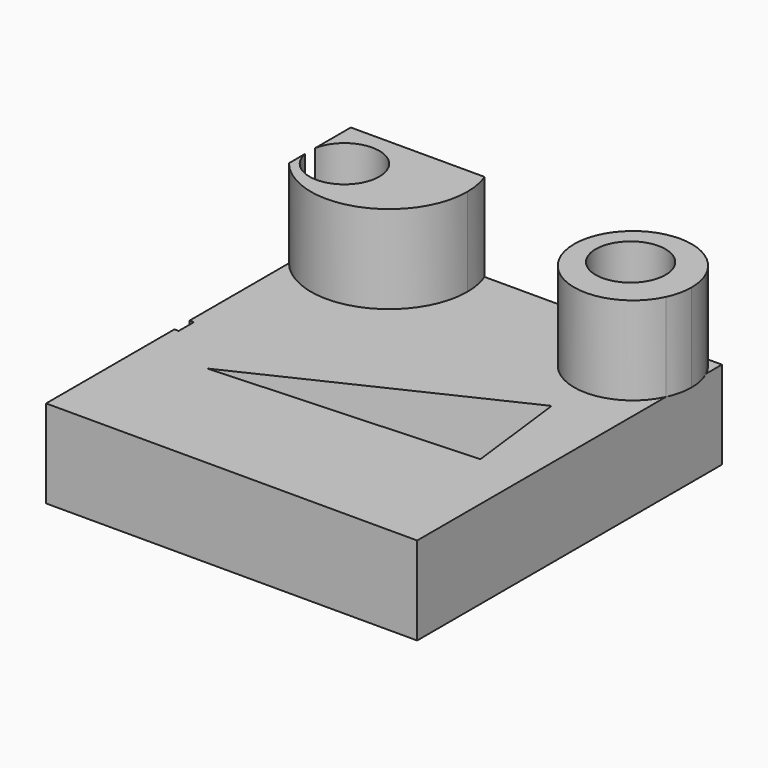
from build123d import *

# Parameters (mm, degrees)
F0_R     = 10.0651181203
F1_DEPTH = 25.4
F2_R     = 10.0651181203
F3_DEPTH = 25.4


with BuildPart() as f1:
    # F0 (on Top) → F1 (new body)
    with BuildSketch(Plane.XY):
        with BuildLine():
            Line((44.1251173615, 55.5551163852), (-62.9092976451, 55.5551163852))
            Line((-62.9092976451, 55.5551163852), (-62.9092976451, 42.5920749035))
            ThreePointArc((-62.9092976451, 42.5920749035), (-52.109599733, 50.8846190086), (-42.9095561607, 40.8467426896))
            ThreePointArc((-42.9095561607, 40.8467426896), (-52.109599733, 30.8088663707), (-62.9092976451, 39.1014104757))
            Line((-62.9092976451, 39.1014104757), (-62.9092976451, -2.5695350487))
            Line((-62.9092976451, -2.5695350487), (-61.6688355803, -2.5695350487))
            Line((-61.6688355803, -2.5695350487), (-61.6688355803, -8.0630239099))
            Line((-61.6688355803, -8.0630239099), (-62.9092976451, -8.0630239099))
            Line((-62.9092976451, -8.0630239099), (-62.9092976451, -54.3146505952))
            Line((-62.9092976451, -54.3146505952), (-55.1120936871, -54.3146505952))
            Line((-55.1120936871, -54.3146505952), (34.910235554, -54.3146505952))
            Line((34.910235554, -54.3146505952), (44.1251173615, -54.3146505952))
            Line((44.1251173615, -54.3146505952), (44.1251173615, 20.8220928907))
            Line((44.1251173615, 20.8220928907), (44.1251173615, 28.4420922399))
            Line((44.1251173615, 28.4420922399), (44.1251173615, 55.5551163852))
        make_face()
        Polygon((30.4799973965, -14.4425584003), (-45.1883710921, -18.3411631733), (26.7586056143, 15.8602334559), align=None, mode=Mode.SUBTRACT)
        with Locations((27.2902306169, 43.6820946634)):
            Circle(F0_R, mode=Mode.SUBTRACT)
    extrude(amount=F1_DEPTH)

    # F2 (on face) → F3 (join)
    with BuildSketch(Plane.XY.offset(25.4)):
        with BuildLine():
            ThreePointArc((-62.9092976451, 33.2274518748), (-37.8353474986, 26.1976296864), (-22.8169896281, 47.4713294781))
            ThreePointArc((-22.8169896281, 47.4713294781), (-23.1943629489, 51.5819332274), (-24.3138670359, 55.5551163852))
            Line((-24.3138670359, 55.5551163852), (-62.9092976451, 55.5551163852))
            Line((-62.9092976451, 55.5551163852), (-62.9092976451, 42.5920749035))
            ThreePointArc((-62.9092976451, 42.5920749035), (-42.9095561607, 40.8467426896), (-62.9092976451, 39.1014104757))
            Line((-62.9092976451, 39.1014104757), (-62.9092976451, 33.2274518748))
        make_face()
        with BuildLine():
            Line((39.7248882397, 55.5551163852), (17.9206636207, 55.5551163852))
            ThreePointArc((17.9206636207, 55.5551163852), (18.4737505401, 29.1833400362), (44.1251173615, 35.3301988385))
            Line((44.1251173615, 35.3301988385), (44.1251173615, 49.8539509685))
            ThreePointArc((44.1251173615, 49.8539509685), (42.2315107975, 52.9411002936), (39.7248882397, 55.5551163852))
        make_face()
        with Locations((27.2902306169, 43.6820946634)):
            Circle(F2_R, mode=Mode.SUBTRACT)
        with BuildLine():
            ThreePointArc((39.7248882397, 55.5551163852), (28.8227759302, 59.5300941875), (17.9206636207, 55.5551163852))
            Line((17.9206636207, 55.5551163852), (39.7248882397, 55.5551163852))
        make_face()
        with BuildLine():
            Line((44.1251173615, 49.8539509685), (44.1251173615, 35.3301988385))
            ThreePointArc((44.1251173615, 35.3301988385), (45.3468167725, 38.8701706187), (45.7607952142, 42.5920749035))
            ThreePointArc((45.7607952142, 42.5920749035), (45.3468167725, 46.3139791883), (44.1251173615, 49.8539509685))
        make_face()
    extrude(amount=F3_DEPTH)


solid = f1.part
